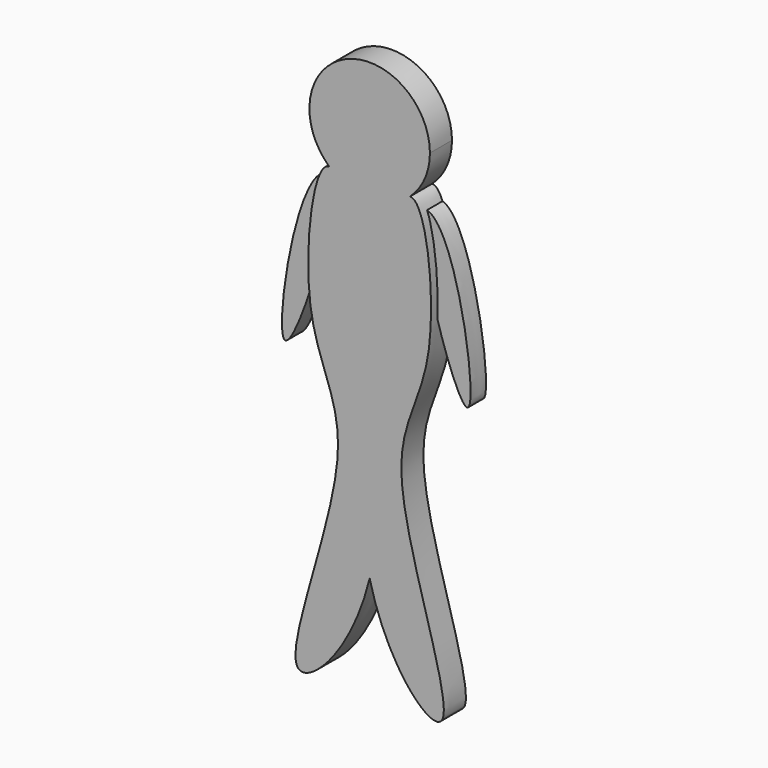
from build123d import *

# Parameters (mm, degrees)
F1_DEPTH = 2.54
F3_DEPTH = 1.778
F5_DEPTH = 3.175


with BuildPart() as f1:
    # F0 (on Front) → F1 (new body)
    with BuildSketch(Plane.XZ):
        with BuildLine():
            ThreePointArc((3.7092103529, 48.7496855453), (5.0671470477, 50.6167193556), (5.5475241636, 52.8748258948))
            ThreePointArc((5.5475241636, 52.8748258948), (-2.2581065392, 57.9419729425), (-3.7092103529, 48.7496855453))
            add(Edge.make_bspline(
                [(-2.9907241633, 48.2025038464), (-3.2397557383, 48.5425687681), (-3.4815269665, 48.7326116248), (-3.7092103529, 48.7496855453)],
                knots=[0.9739839009, 0.9739839009, 0.9739839009, 0.9739839009, 1, 1, 1, 1], degree=3))
            ThreePointArc((-2.9907241633, 48.2025038464), (0, 47.3273017313), (2.9907241633, 48.2025038464))
            add(Edge.make_bspline(
                [(2.9907241633, 48.2025038464), (3.2397557383, 48.5425687681), (3.4815269665, 48.7326116248), (3.7092103529, 48.7496855453)],
                knots=[0.9739839009, 0.9739839009, 0.9739839009, 0.9739839009, 1, 1, 1, 1], degree=3))
        make_face()
        with BuildLine():
            add(Edge.make_bspline(
                [(-2.9907241633, 48.2025038464), (-3.2397557383, 48.5425687681), (-3.4815269665, 48.7326116248), (-3.7092103529, 48.7496855453)],
                knots=[0.9739839009, 0.9739839009, 0.9739839009, 0.9739839009, 1, 1, 1, 1], degree=3))
            ThreePointArc((-3.7092103529, 48.7496855453), (-3.3611207332, 48.4614494366), (-2.9907241633, 48.2025038464))
        make_face()
        with BuildLine():
            ThreePointArc((-2.9907241633, 48.2025038464), (-3.3611207332, 48.4614494366), (-3.7092103529, 48.7496855453))
            add(Edge.make_bspline(
                [(-3.7092103529, 48.7496855453), (-5.2134349849, 48.8624869767), (-6.9665224437, 34.2023470282), (0.0869990049, 27.7907233929), (-11.1463797548, 0.9426416028), (-1.6939504177, 9.6754793133), (0, 16.5912210941)],
                knots=[0, 0, 0, 0, 0.1718792822, 0.3388196933, 0.5521260112, 0.719135411, 0.719135411, 0.719135411, 0.719135411], degree=3))
            add(Edge.make_bspline(
                [(0, 16.5912210941), (-1.4883559473, 22.6676004864), (-1.0799851415, 31.1223756669), (0, 37.8380047216)],
                knots=[0.719135411, 0.719135411, 0.719135411, 0.719135411, 0.8658749087, 0.8658749087, 0.8658749087, 0.8658749087], degree=3))
            add(Edge.make_bspline(
                [(0, 37.8380047216), (-0.7956692442, 42.7856834341), (-1.9558821397, 46.7893759257), (-2.9907241633, 48.2025038464)],
                knots=[0.8658749087, 0.8658749087, 0.8658749087, 0.8658749087, 0.9739839009, 0.9739839009, 0.9739839009, 0.9739839009], degree=3))
        make_face()
        with BuildLine():
            add(Edge.make_bspline(
                [(3.7092103529, 48.7496855453), (5.2134349849, 48.8624869767), (6.9665224437, 34.2023470282), (-0.0869990049, 27.7907233929), (11.1463797548, 0.9426416028), (1.6939504177, 9.6754793133), (0, 16.5912210941)],
                knots=[0, 0, 0, 0, 0.1718792822, 0.3388196933, 0.5521260112, 0.719135411, 0.719135411, 0.719135411, 0.719135411], degree=3))
            ThreePointArc((3.7092103529, 48.7496855453), (3.3611207332, 48.4614494366), (2.9907241633, 48.2025038464))
            add(Edge.make_bspline(
                [(0, 37.8380047216), (0.7956692442, 42.7856834341), (1.9558821397, 46.7893759257), (2.9907241633, 48.2025038464)],
                knots=[0.8658749087, 0.8658749087, 0.8658749087, 0.8658749087, 0.9739839009, 0.9739839009, 0.9739839009, 0.9739839009], degree=3))
            add(Edge.make_bspline(
                [(0, 16.5912210941), (1.4883559473, 22.6676004864), (1.0799851415, 31.1223756669), (0, 37.8380047216)],
                knots=[0.719135411, 0.719135411, 0.719135411, 0.719135411, 0.8658749087, 0.8658749087, 0.8658749087, 0.8658749087], degree=3))
        make_face()
        with BuildLine():
            ThreePointArc((2.9907241633, 48.2025038464), (3.3611207332, 48.4614494366), (3.7092103529, 48.7496855453))
            add(Edge.make_bspline(
                [(2.9907241633, 48.2025038464), (3.2397557383, 48.5425687681), (3.4815269665, 48.7326116248), (3.7092103529, 48.7496855453)],
                knots=[0.9739839009, 0.9739839009, 0.9739839009, 0.9739839009, 1, 1, 1, 1], degree=3))
        make_face()
        with BuildLine():
            ThreePointArc((2.9907241633, 48.2025038464), (0, 47.3273017313), (-2.9907241633, 48.2025038464))
            add(Edge.make_bspline(
                [(0, 37.8380047216), (-0.7956692442, 42.7856834341), (-1.9558821397, 46.7893759257), (-2.9907241633, 48.2025038464)],
                knots=[0.8658749087, 0.8658749087, 0.8658749087, 0.8658749087, 0.9739839009, 0.9739839009, 0.9739839009, 0.9739839009], degree=3))
            add(Edge.make_bspline(
                [(0, 37.8380047216), (0.7956692442, 42.7856834341), (1.9558821397, 46.7893759257), (2.9907241633, 48.2025038464)],
                knots=[0.8658749087, 0.8658749087, 0.8658749087, 0.8658749087, 0.9739839009, 0.9739839009, 0.9739839009, 0.9739839009], degree=3))
        make_face()
        with BuildLine():
            add(Edge.make_bspline(
                [(0, 16.5912210941), (-1.4883559473, 22.6676004864), (-1.0799851415, 31.1223756669), (0, 37.8380047216)],
                knots=[0.719135411, 0.719135411, 0.719135411, 0.719135411, 0.8658749087, 0.8658749087, 0.8658749087, 0.8658749087], degree=3))
            add(Edge.make_bspline(
                [(0, 16.5912210941), (1.4883559473, 22.6676004864), (1.0799851415, 31.1223756669), (0, 37.8380047216)],
                knots=[0.719135411, 0.719135411, 0.719135411, 0.719135411, 0.8658749087, 0.8658749087, 0.8658749087, 0.8658749087], degree=3))
        make_face()
    extrude(amount=F1_DEPTH)

    # F2 (on Front) → F3 (join)
    with BuildSketch(Plane.XZ):
        with BuildLine():
            add(Edge.make_bspline(
                [(-2.9766794036, 46.5529243472), (-2.81037839, 47.0855158144), (-6.8678972042, 50.8395924164), (-11.0141828945, 22.0518304425), (-3.4722826714, 44.7214617456), (-5.4643228295, 45.9482695744), (-3.1316790274, 46.0565264283), (-2.9766794036, 46.5529243472)],
                knots=[0, 0, 0, 0, 0.1299325031, 0.4708050688, 0.7779578337, 0.8788973761, 1, 1, 1, 1], degree=3))
        make_face()
        with BuildLine():
            add(Edge.make_bspline(
                [(2.9766794036, 46.5529243472), (2.81037839, 47.0855158144), (6.8678972042, 50.8395924164), (11.0141828945, 22.0518304425), (3.4722826714, 44.7214617456), (5.4643228295, 45.9482695744), (3.1316790274, 46.0565264283), (2.9766794036, 46.5529243472)],
                knots=[0, 0, 0, 0, 0.1299325031, 0.4708050688, 0.7779578337, 0.8788973761, 1, 1, 1, 1], degree=3))
        make_face()
    extrude(amount=F3_DEPTH)


with BuildPart() as f5:
    # F4 (on Front) → F5 (new body)
    with BuildSketch(Plane.XZ):
        with BuildLine():
            add(Edge.make_bspline(
                [(0, 43.0366061628), (0.8643144804, 44.4003418497), (1.6647448264, 46.9773033289), (0, 49.4899712503)],
                knots=[0.943280188, 0.943280188, 0.943280188, 0.943280188, 1, 1, 1, 1], degree=3))
            add(Edge.make_bspline(
                [(0, 43.0366061628), (-0.8643144804, 44.4003418497), (-1.6647448264, 46.9773033289), (0, 49.4899712503)],
                knots=[0.943280188, 0.943280188, 0.943280188, 0.943280188, 1, 1, 1, 1], degree=3))
        make_face()
        with BuildLine():
            add(Edge.make_bspline(
                [(0, 43.0366061628), (-0.8643144804, 44.4003418497), (-1.6647448264, 46.9773033289), (0, 49.4899712503)],
                knots=[0.943280188, 0.943280188, 0.943280188, 0.943280188, 1, 1, 1, 1], degree=3))
            add(Edge.make_bspline(
                [(0, 49.4899712503), (-2.2231687437, 52.8454913862), (-19.4626691015, 61.2857358657), (-2.5319177673, 4.3203098968), (-11.5812345835, 50.1351195221), (-3.4298269541, 14.1483642287), (-9.341972182, 49.4482532476), (-1.2007033383, 12.5482912672), (-7.9621154493, 49.231769969), (-0.0993578774, 17.6327924998), (-5.937169, 48.9375203474), (0.858972439, 16.2878370844), (-2.6565717905, 41.0508920763), (-0.6658187024, 41.9860617765), (0, 43.0366061628)],
                knots=[0, 0, 0, 0, 0.0757459709, 0.1972670057, 0.2828141129, 0.3605634713, 0.4371862329, 0.5170303649, 0.597274528, 0.6697995602, 0.7425321953, 0.8196767058, 0.8995864718, 0.943280188, 0.943280188, 0.943280188, 0.943280188], degree=3))
        make_face()
        with BuildLine():
            add(Edge.make_bspline(
                [(0, 49.4899712503), (2.2231687437, 52.8454913862), (19.4626691015, 61.2857358657), (2.5319177673, 4.3203098968), (11.5812345835, 50.1351195221), (3.4298269541, 14.1483642287), (9.341972182, 49.4482532476), (1.2007033383, 12.5482912672), (7.9621154493, 49.231769969), (0.0993578774, 17.6327924998), (5.937169, 48.9375203474), (-0.858972439, 16.2878370844), (2.6565717905, 41.0508920763), (0.6658187024, 41.9860617765), (0, 43.0366061628)],
                knots=[0, 0, 0, 0, 0.0757459709, 0.1972670057, 0.2828141129, 0.3605634713, 0.4371862329, 0.5170303649, 0.597274528, 0.6697995602, 0.7425321953, 0.8196767058, 0.8995864718, 0.943280188, 0.943280188, 0.943280188, 0.943280188], degree=3))
            add(Edge.make_bspline(
                [(0, 43.0366061628), (0.8643144804, 44.4003418497), (1.6647448264, 46.9773033289), (0, 49.4899712503)],
                knots=[0.943280188, 0.943280188, 0.943280188, 0.943280188, 1, 1, 1, 1], degree=3))
        make_face()
    extrude(amount=-F5_DEPTH)


solid = f1.part
